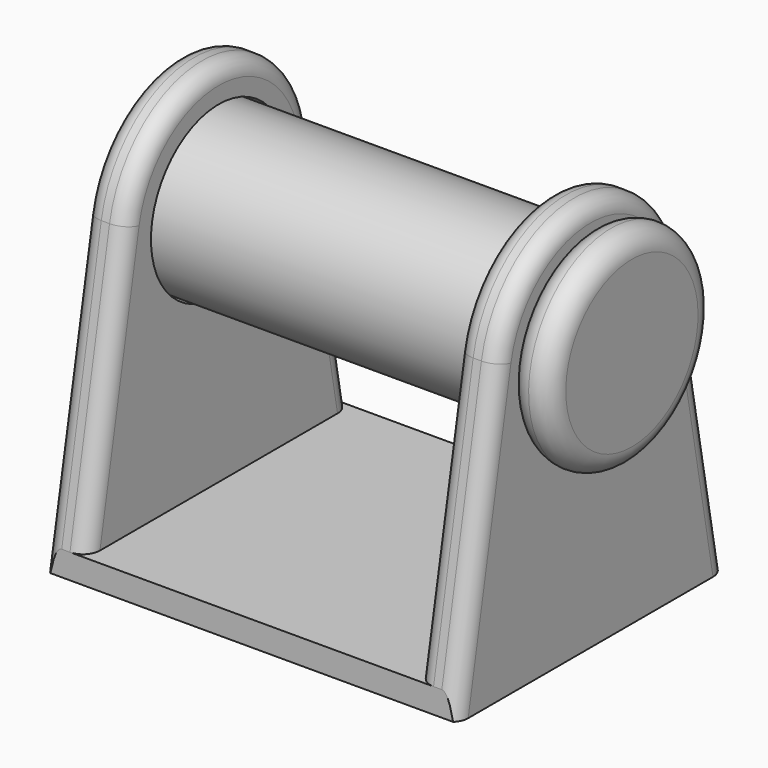
from build123d import *

# Parameters (mm, degrees)
F0_W     = 40
F0_H     = 40
F0_W_2   = 5
F1_DEPTH = 3
F3_START = 20
F2_R     = 10.25
F3_DEPTH = 5
F4_START = -20
F4_DEPTH = 5
F5_W     = 50
F5_H     = 10
F7_R     = 2
F8_R     = 2.49999
F9_SIZE  = 1


# Not quite as in the source:
# - a fillet or chamfer is up to 0.001 mm smaller than in the source, because OpenCascade refuses the exact size


with BuildPart() as f1:
    # F0 (on Top) → F1 (new body)
    with BuildSketch(Plane.XY):
        Rectangle(F0_W, F0_H)
        with Locations((-22.5, 0)):
            Rectangle(F0_W_2, F0_H)
        with Locations((22.5, 0)):
            Rectangle(F0_W_2, F0_H)
    extrude(amount=F1_DEPTH)

    # F2 (on Right) → F3 (join)
    with BuildSketch(Plane.YZ.offset(F3_START)):
        with BuildLine():
            ThreePointArc((14.0154384668, 35.5748756445), (14.1912384617, 34.2927687049), (14.25, 33))
            ThreePointArc((14.25, 33), (-1.2927687049, 18.8087615383), (-14.0154384668, 35.5748756445))
            Line((-14.0154384668, 35.5748756445), (-20, 3))
            Line((-20, 3), (20, 3))
            Line((20, 3), (14.0154384668, 35.5748756445))
        make_face()
        with BuildLine():
            ThreePointArc((-14.0154384668, 35.5748756445), (-1.2927687049, 18.8087615383), (14.25, 33))
            ThreePointArc((14.25, 33), (14.1912384617, 34.2927687049), (14.0154384668, 35.5748756445))
            ThreePointArc((14.0154384668, 35.5748756445), (0, 47.25), (-14.0154384668, 35.5748756445))
        make_face()
        with Locations((0, 33)):
            Circle(F2_R, mode=Mode.SUBTRACT)
    extrude(amount=F3_DEPTH)

    # F2 (on Right) → F4 (join)
    with BuildSketch(Plane.YZ.offset(F4_START)):
        with BuildLine():
            ThreePointArc((14.0154384668, 35.5748756445), (14.1912384617, 34.2927687049), (14.25, 33))
            ThreePointArc((14.25, 33), (-1.2927687049, 18.8087615383), (-14.0154384668, 35.5748756445))
            Line((-14.0154384668, 35.5748756445), (-20, 3))
            Line((-20, 3), (20, 3))
            Line((20, 3), (14.0154384668, 35.5748756445))
        make_face()
        with BuildLine():
            ThreePointArc((-14.0154384668, 35.5748756445), (-1.2927687049, 18.8087615383), (14.25, 33))
            ThreePointArc((14.25, 33), (14.1912384617, 34.2927687049), (14.0154384668, 35.5748756445))
            ThreePointArc((14.0154384668, 35.5748756445), (0, 47.25), (-14.0154384668, 35.5748756445))
        make_face()
        with Locations((0, 33)):
            Circle(F2_R, mode=Mode.SUBTRACT)
    extrude(amount=-F4_DEPTH)

    # F7
    f7_edges = [f1.edges().sort_by_distance(p)[0] for p in [
        (-20, 17.007719, 19.287438),
        (-25, 17.007719, 19.287438),
        (20, 17.007719, 19.287438),
        (25, 17.007719, 19.287438),
    ]]
    fillet(f7_edges, radius=F7_R)


with BuildPart() as f6:
    # F5 (on Front) → F6 (revolve)
    with BuildSketch(Plane.XZ):
        with Locations((0, 28)):
            Rectangle(F5_W, F5_H)
        Polygon((25, 33), (25, 23), (25, 20.5), (30, 20.5), (30, 33), align=None)
    revolve(axis=Axis((0, 0, 33), (-1, 0, 0)))

    # F8 (radius 2.5 in the source; OpenCascade refuses exactly that, so slightly less here)
    f8_edges = [f6.edges().sort_by_distance(p)[0] for p in [
        (30, 0, 45.5),
        (25, 0, 45.5),
    ]]
    fillet(f8_edges, radius=F8_R)

    # F9
    f9_edges = [f6.edges().sort_by_distance(p)[0] for p in [
        (-25, 0, 43),
    ]]
    chamfer(f9_edges, length=F9_SIZE)


solid = Compound([f1.part, f6.part])
